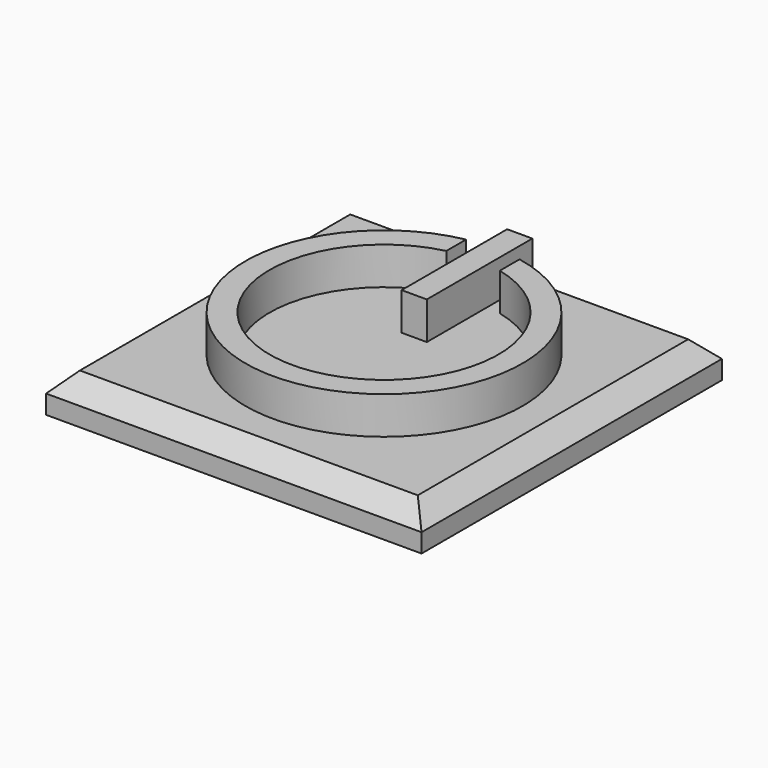
from build123d import *

# Parameters (mm, degrees)
F0_W         = 100
F0_H         = 100
F1_DEPTH     = 10
F2_W         = 6.7138946615
F2_H         = 35.1261794567
F3_DEPTH     = 10
F4_T1_DEPTH  = 125.7168298797
F4_T3_DEPTH  = 125.7168298797
F4_T8_DEPTH  = 125.7168298797
F4_T14_DEPTH = 125.7168298797
F4_T20_DEPTH = 125.7168298797
F4_T27_DEPTH = 125.7168298797
F4_T33_DEPTH = 125.7168298797
F5_TEXT_SIZE = 22.3098133118
F6_DEPTH     = 5


# Not quite as in the source:
# - a fillet or chamfer that OpenCascade refuses, or shapes differently, is made with other operations: its cross-section is extruded or revolved along the edge and cut away or added
# - Text() gives the source's letters only with a copy of the font that has no kerning and outlines rounded to 1/6400 em; it was checked with that copy


with BuildPart() as f1:
    # F0 (on Top) → F1 (new body)
    with BuildSketch(Plane.XY):
        Rectangle(F0_W, F0_H)
    extrude(amount=F1_DEPTH)

    # F2 (on face) → F3 (join)
    with BuildSketch(Plane.XY.offset(10)):
        with BuildLine():
            Line((-7.1218120866, 29.64928665), (-7.1218120866, 36.2191033053))
            ThreePointArc((-7.1218120866, 36.2191033053), (0, -36.9126489382), (7.1218120866, 36.2191033053))
            Line((7.1218120866, 36.2191033053), (7.1218120866, 29.64928665))
            ThreePointArc((7.1218120866, 29.64928665), (0, -30.4926287199), (-7.1218120866, 29.64928665))
        make_face()
        with Locations((0, 27.6284813881)):
            Rectangle(F2_W, F2_H)
    extrude(amount=F3_DEPTH)

    # F4: chamfer of 5 on 4 edges, made by hand

    # F4_s2 → F4_t1 (cut)
    with BuildSketch(Plane.XZ.offset(-62.8584149398)):
        Polygon((-50, 5), (-45, 10), (-50, 10), align=None)
        Polygon((50, 5), (45, 10), (50, 10), align=None)
    extrude(amount=F4_T1_DEPTH, mode=Mode.SUBTRACT)

    # F4_s4 → F4_t3 (cut)
    with BuildSketch(Plane.YZ.offset(-62.8584149398)):
        Polygon((-45, 10), (-50, 5), (-50, 10), align=None)
    extrude(amount=F4_T3_DEPTH, mode=Mode.SUBTRACT)


with BuildPart() as f4_tool6:
    # F4_s7 → F4_t8 (new body)
    with BuildSketch(Plane.YZ.offset(62.8584149398)):
        Polygon((50, 5), (45, 10), (50, 10), align=None)
    extrude(amount=-F4_T8_DEPTH)

    split(bisect_by=Plane.YZ.offset(3.3569473308), keep=Keep.TOP)

    split(bisect_by=Plane.XZ.offset(-45.1915711164), keep=Keep.BOTTOM)


with BuildPart() as f1_1:
    add(f1.part)

    # F4_t5: cut F4_tool6
    add(f4_tool6.part, mode=Mode.SUBTRACT)


with BuildPart() as f4_tool12:
    # F4_s13 → F4_t14 (new body)
    with BuildSketch(Plane.YZ.offset(62.8584149398)):
        Polygon((50, 5), (45, 10), (50, 10), align=None)
    extrude(amount=-F4_T14_DEPTH)

    split(bisect_by=Plane.YZ.offset(3.3569473308), keep=Keep.TOP)

    split(bisect_by=Plane.XZ.offset(-45.1915711164), keep=Keep.TOP)


with BuildPart() as f1_2:
    add(f1_1.part)

    # F4_t11: cut F4_tool12
    add(f4_tool12.part, mode=Mode.SUBTRACT)


with BuildPart() as f4_tool18:
    # F4_s19 → F4_t20 (new body)
    with BuildSketch(Plane.YZ.offset(62.8584149398)):
        Polygon((50, 5), (45, 10), (50, 10), align=None)
    extrude(amount=-F4_T20_DEPTH)

    split(bisect_by=Plane.YZ.offset(-3.3569473308), keep=Keep.TOP)

    split(bisect_by=Plane.YZ.offset(3.3569473308), keep=Keep.BOTTOM)

    split(bisect_by=Plane.XZ.offset(-45.1915711164), keep=Keep.BOTTOM)


with BuildPart() as f1_3:
    add(f1_2.part)

    # F4_t17: cut F4_tool18
    add(f4_tool18.part, mode=Mode.SUBTRACT)


with BuildPart() as f4_tool25:
    # F4_s26 → F4_t27 (new body)
    with BuildSketch(Plane.YZ.offset(62.8584149398)):
        Polygon((50, 5), (45, 10), (50, 10), align=None)
    extrude(amount=-F4_T27_DEPTH)

    split(bisect_by=Plane.YZ.offset(-3.3569473308), keep=Keep.BOTTOM)

    split(bisect_by=Plane.XZ.offset(-45.1915711164), keep=Keep.BOTTOM)


with BuildPart() as f1_4:
    add(f1_3.part)

    # F4_t24: cut F4_tool25
    add(f4_tool25.part, mode=Mode.SUBTRACT)


with BuildPart() as f4_tool31:
    # F4_s32 → F4_t33 (new body)
    with BuildSketch(Plane.YZ.offset(62.8584149398)):
        Polygon((50, 5), (45, 10), (50, 10), align=None)
    extrude(amount=-F4_T33_DEPTH)

    split(bisect_by=Plane.YZ.offset(-3.3569473308), keep=Keep.BOTTOM)

    split(bisect_by=Plane.XZ.offset(-45.1915711164), keep=Keep.TOP)


with BuildPart() as f1_5:
    add(f1_4.part)

    # F4_t30: cut F4_tool31
    add(f4_tool31.part, mode=Mode.SUBTRACT)

    # F5 (on face) → F6 (cut)
    with BuildSketch(Plane(origin=(0, 0, 0), x_dir=(1, 0, 0), z_dir=(0, 0, -1))):
        with Locations((-39.5755172702, -8.0315327923)):
            Text('BY A.G.', F5_TEXT_SIZE, font='Open Sans', font_style=FontStyle.BOLD, text_align=(TextAlign.LEFT, TextAlign.BOTTOM))
    extrude(amount=-F6_DEPTH, mode=Mode.SUBTRACT)


solid = f1_5.part
